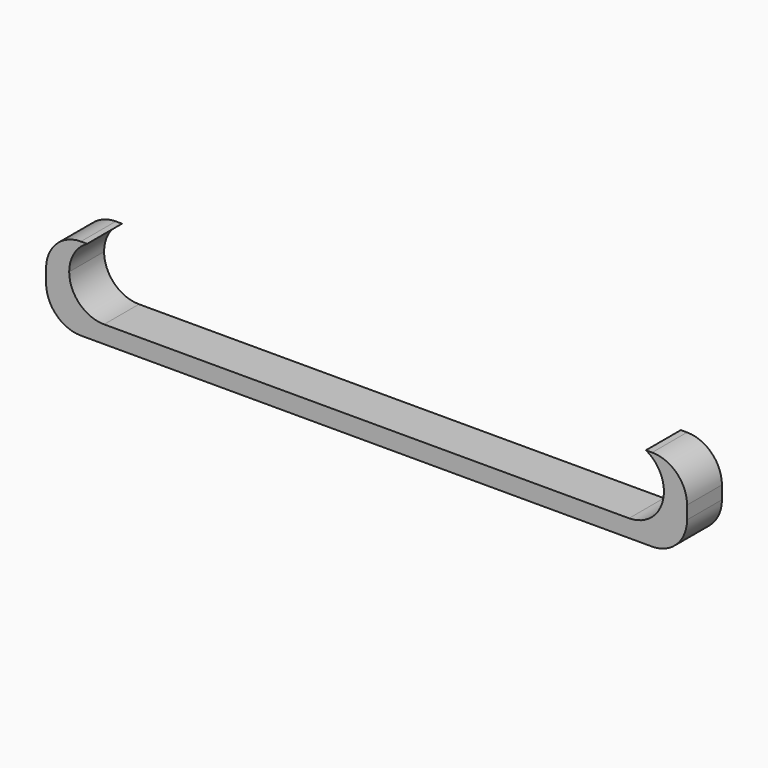
from build123d import *

# Parameters (mm, degrees)
F0_W     = 73.5
F0_H     = 5
F1_DEPTH = 10
F2_W     = 68.2
F2_H     = 5
F3_DEPTH = 8
F4_R     = 4
F5_DEPTH = 2
F6_W     = 5
F6_H     = 2
F7_DEPTH = 76.5
F8_R     = 3.99999
F9_DEPTH = 2.5
F10_R    = 4


# Not quite as in the source:
# - a fillet or chamfer is up to 0.001 mm smaller than in the source, because OpenCascade refuses the exact size


with BuildPart() as f1:
    # F0 (on Top) → F1 (new body)
    with BuildSketch(Plane.XY):
        Rectangle(F0_W, F0_H)
    extrude(amount=F1_DEPTH)

    # F2 (on face) → F3 (cut)
    with BuildSketch(Plane.XY.offset(10)):
        Rectangle(F2_W, F2_H)
    extrude(amount=-F3_DEPTH, mode=Mode.SUBTRACT)

    # F4
    f4_edges = [f1.edges().sort_by_distance(p)[0] for p in [
        (34.1, 0, 2),
        (-34.1, 0, 2),
    ]]
    fillet(f4_edges, radius=F4_R)

    # F5 (add): a face of the model
    f5_faces = [f1.faces().sort_by_distance(p)[0] for p in [
        (-35.425, 0, 10),
    ]]
    extrude(f5_faces, amount=F5_DEPTH)

    # F6 (on face) → F7 (join)
    with BuildSketch(Plane.YZ.offset(-34.1)):
        with Locations((0, 11)):
            Rectangle(F6_W, F6_H)
    extrude(amount=F7_DEPTH)

    # F8 (radius 4 in the source; OpenCascade refuses exactly that, so slightly less here)
    f8_edges = [f1.edges().sort_by_distance(p)[0] for p in [
        (-34.1, 0, 10),
        (34.1, 0, 10),
    ]]
    fillet(f8_edges, radius=F8_R)

    # F9 (cut): a face of the model
    f9_faces = [f1.faces().sort_by_distance(p)[0] for p in [
        (2.825, 0, 12),
    ]]
    extrude(f9_faces, amount=-F9_DEPTH, mode=Mode.SUBTRACT)

    # F10
    f10_edges = [f1.edges().sort_by_distance(p)[0] for p in [
        (36.75, 0, 0),
        (-36.75, 0, 9.5),
        (-36.75, 0, 0),
        (36.75, 0, 9.5),
    ]]
    fillet(f10_edges, radius=F10_R)


solid = f1.part
